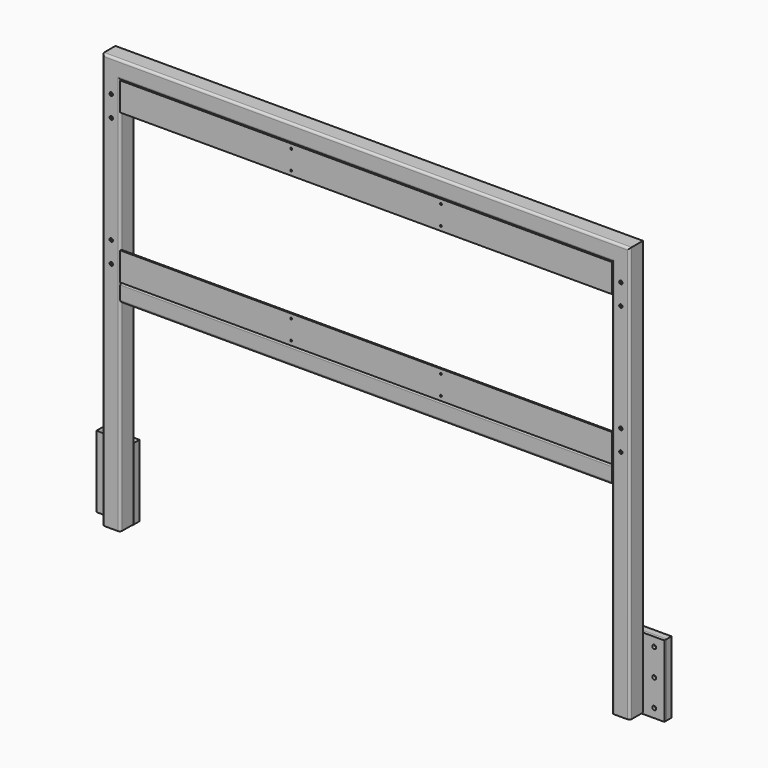
from build123d import *

# Parameters (mm, degrees)
F0_W      = 152.4
F0_H      = 304.8
F1_DEPTH  = 25.4
F3_D      = 13.49248
F4_W      = 152.4
F4_H      = 304.8
F5_DEPTH  = 12.7
F6_D      = 16.66748
F15_W     = 57.15
F15_H     = 4.7625
F16_DEPTH = 2089.404
F17_W     = 6
F17_H     = 120
F18_DEPTH = 2089.404
F20_D     = 8
F20_2_D   = 8
F22_D     = 14.2875


# Not quite as in the source:
# - a length typed as a fraction of an inch, garbled in the dataset ("3 / 203.2 mm" for 3/8 in), is restored


with BuildPart() as f1:
    # F0 (on Front) → F1 (new body)
    with BuildSketch(Plane.XZ):
        with Locations((1130.427, -46.7093307734)):
            Rectangle(F0_W, F0_H)
    extrude(amount=-F1_DEPTH)

    # F3 (through all)
    with Locations(Plane.XZ):
        with Locations((1163.701, 67.5906692266), (1163.701, -46.7093307734), (1163.701, -161.0093307734)):
            Hole(F3_D / 2)


with BuildPart() as f5:
    # F4 (on face) → F5 (new body)
    with BuildSketch(Plane.XZ):
        with Locations((1130.427, -46.7093307734)):
            Rectangle(F4_W, F4_H)
    extrude(amount=F5_DEPTH)

    # F6 (through all)
    with Locations(Plane(origin=(0, 0, 0), x_dir=(1, 0, 0), z_dir=(0, 1, 0))):
        with Locations((1163.701, -67.5906692266), (1163.701, 46.7093307734), (1163.701, 161.0093307734)):
            Hole(F6_D / 2)


with BuildPart() as f7_1:
    # F7: instance of F1
    add(f1.part.mirror(Plane.YZ))


with BuildPart() as f7_2:
    # F7: instance of F5
    add(f5.part.mirror(Plane.YZ))


with BuildPart() as f12:
    # F12: sweep along a path in F9
    with BuildLine(Plane.XZ.offset(50.8)) as f12_path:
        Line((-1082.802, -189.5843307734), (-1082.802, 1537.6156692266))
        Line((-1082.802, 1537.6156692266), (1082.802, 1537.6156692266))
        Line((1082.802, 1537.6156692266), (1082.802, -189.5843307734))
    # F11 (on offset) → F12 (sweep)
    with BuildSketch(Plane(origin=(0, 0, -189.5843307734), x_dir=(1, 0, 0), z_dir=(0, 0, -1))):
        with BuildLine():
            Line((-1054.227, 88.9), (-1111.377, 88.9))
            ThreePointArc((-1111.377, 88.9), (-1118.1121920908, 86.1101920908), (-1120.902, 79.375))
            Line((-1120.902, 79.375), (-1120.902, 22.225))
            ThreePointArc((-1120.902, 22.225), (-1118.1121920908, 15.4898079092), (-1111.377, 12.7))
            Line((-1111.377, 12.7), (-1054.227, 12.7))
            ThreePointArc((-1054.227, 12.7), (-1047.4918079092, 15.4898079092), (-1044.702, 22.225))
            Line((-1044.702, 22.225), (-1044.702, 79.375))
            ThreePointArc((-1044.702, 79.375), (-1047.4918079092, 86.1101920908), (-1054.227, 88.9))
        make_face()
        with BuildLine():
            ThreePointArc((-1114.552, 79.375), (-1113.6220640303, 81.6200640303), (-1111.377, 82.55))
            Line((-1111.377, 82.55), (-1054.227, 82.55))
            ThreePointArc((-1054.227, 82.55), (-1051.9819359697, 81.6200640303), (-1051.052, 79.375))
            Line((-1051.052, 79.375), (-1051.052, 22.225))
            ThreePointArc((-1051.052, 22.225), (-1051.9819359697, 19.9799359697), (-1054.227, 19.05))
            Line((-1054.227, 19.05), (-1111.377, 19.05))
            ThreePointArc((-1111.377, 19.05), (-1113.6220640303, 19.9799359697), (-1114.552, 22.225))
            Line((-1114.552, 22.225), (-1114.552, 79.375))
        make_face(mode=Mode.SUBTRACT)
    sweep(path=f12_path.line, transition=Transition.RIGHT)

    # F15 (on face) → F16 (join, through all)
    with BuildSketch(Plane.YZ.offset(-1044.702)):
        with BuildLine():
            Line((-79.375, 739.1158692266), (-79.375, 743.8783692266))
            ThreePointArc((-79.375, 743.8783692266), (-86.1101920908, 741.0885613174), (-88.9, 734.3533692266))
            Line((-88.9, 734.3533692266), (-88.9, 677.2033692266))
            ThreePointArc((-88.9, 677.2033692266), (-86.1101920908, 670.4681771358), (-79.375, 667.6783692266))
            Line((-79.375, 667.6783692266), (-79.375, 672.4408692266))
            ThreePointArc((-79.375, 672.4408692266), (-82.7425960454, 673.8357731812), (-84.1375, 677.2033692266))
            Line((-84.1375, 677.2033692266), (-84.1375, 734.3533692266))
            ThreePointArc((-84.1375, 734.3533692266), (-82.7425960454, 737.720965272), (-79.375, 739.1158692266))
        make_face()
        with Locations((-50.8, 741.4971192266)):
            Rectangle(F15_W, F15_H)
        with BuildLine():
            ThreePointArc((-12.7, 734.3533692266), (-15.4898079092, 741.0885613174), (-22.225, 743.8783692266))
            Line((-22.225, 743.8783692266), (-22.225, 739.1158692266))
            ThreePointArc((-22.225, 739.1158692266), (-18.8574039546, 737.720965272), (-17.4625, 734.3533692266))
            Line((-17.4625, 734.3533692266), (-17.4625, 677.2033692266))
            ThreePointArc((-17.4625, 677.2033692266), (-18.8574039546, 673.8357731812), (-22.225, 672.4408692266))
            Line((-22.225, 672.4408692266), (-22.225, 667.6783692266))
            ThreePointArc((-22.225, 667.6783692266), (-15.4898079092, 670.4681771358), (-12.7, 677.2033692266))
            Line((-12.7, 677.2033692266), (-12.7, 734.3533692266))
        make_face()
        with Locations((-50.8, 670.0596192266)):
            Rectangle(F15_W, F15_H)
    extrude(amount=F16_DEPTH)

    # F22 (through all)
    with Locations(Plane.XZ.offset(88.9)):
        with Locations((-1082.802, 1436.0156692266), (-1082.802, 1347.1156692266), (-1082.802, 889.9156692266), (-1082.802, 801.0156692266), (1082.802, 1436.0156692266), (1082.802, 1347.1156692266), (1082.802, 889.9156692266), (1082.802, 801.0156692266)):
            Hole(F22_D / 2)


with BuildPart() as f18:
    # F17 (on face) → F18 (new body, through all)
    with BuildSketch(Plane(origin=(1044.702, 0, 0), x_dir=(0, -1, 0), z_dir=(-1, 0, 0))):
        with Locations((85.9, 1439.5156692266)):
            Rectangle(F17_W, F17_H)
    extrude(amount=F18_DEPTH)

    # F20 (through all)
    with Locations(Plane.XZ.offset(88.9)):
        with Locations((-318, 844.8783692266), (-318, 762.8783692266), (318, 844.8783692266), (318, 762.8783692266), (-318, 1480.5156692266), (-318, 1398.5156692266), (318, 1480.5156692266), (318, 1398.5156692266)):
            Hole(F20_D / 2)


with BuildPart() as f18b:
    # F17 (on face) → F18, piece 2 (new body, through all)
    with BuildSketch(Plane(origin=(1044.702, 0, 0), x_dir=(0, -1, 0), z_dir=(-1, 0, 0))):
        with Locations((85.9, 803.8783692266)):
            Rectangle(F17_W, F17_H)
    extrude(amount=F18_DEPTH)

    # F20#2 (through all)
    with Locations(Plane.XZ.offset(88.9)):
        with Locations((-318, 844.8783692266), (-318, 762.8783692266), (318, 844.8783692266), (318, 762.8783692266), (-318, 1480.5156692266), (-318, 1398.5156692266), (318, 1480.5156692266), (318, 1398.5156692266)):
            Hole(F20_2_D / 2)


solid = Compound([f1.part, f5.part, f7_1.part, f7_2.part, f12.part, f18.part, f18b.part])
